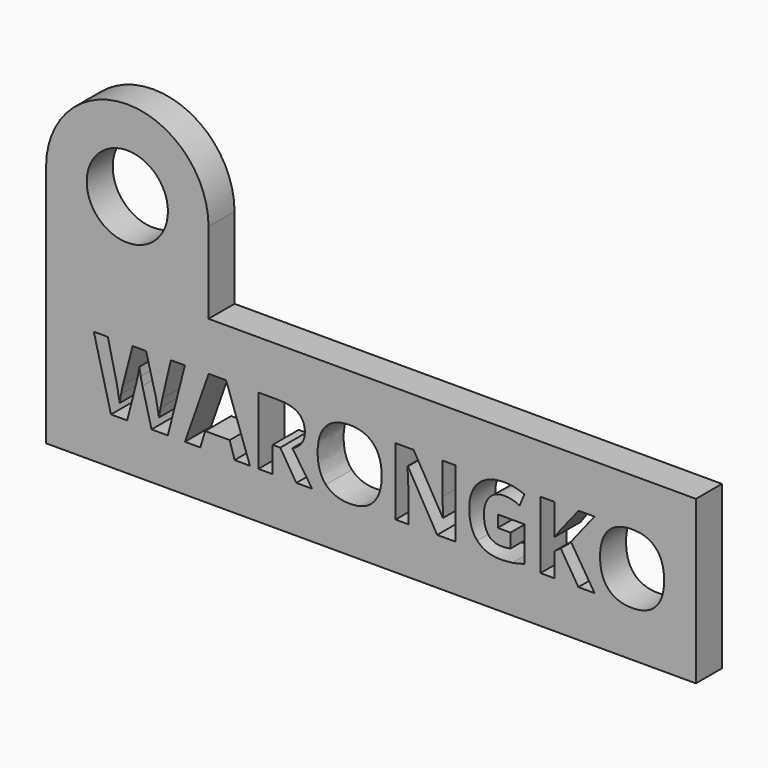
from build123d import *

# Parameters (mm, degrees)
F0_R     = 6.35
F1_DEPTH = 5.08
F2_DEPTH = 25.4


# Not quite as in the source:
# - a feature names something its author has since deleted; it is built from what else it names


with BuildPart() as f1:
    # F0 (on Front) → F1 (new body)
    with BuildSketch(Plane.XZ):
        with BuildLine():
            ThreePointArc((25.4, 38.1), (12.7, 50.8), (0, 38.1))
            ThreePointArc((0, 38.1), (12.7, 25.4), (25.4, 38.1))
        make_face()
        with Locations((12.7, 38.1)):
            Circle(F0_R, mode=Mode.SUBTRACT)
        with BuildLine():
            Line((0, 38.1), (0, 0))
            Line((0, 0), (12.7, 0))
            Line((12.7, 0), (50.8, 0))
            Line((50.8, 0), (101.6, 0))
            Line((101.6, 0), (101.6, 25.4))
            Line((101.6, 25.4), (25.4, 25.4))
            Line((25.4, 25.4), (25.4, 38.1))
            ThreePointArc((25.4, 38.1), (12.7, 25.4), (0, 38.1))
        make_face()
        with BuildLine():
            Line((21.7064113992, 17.7952383145), (19.0291020371, 7.2770728152))
            Line((19.0291020371, 7.2770728152), (16.4899169757, 7.2770728152))
            Line((16.4899169757, 7.2770728152), (15.0649346066, 12.8020448437))
            add(Edge.make_bspline(
                [(15.0649346066, 12.8020448437), (14.9866641696, 13.0967100185), (14.7955922203, 14.0209917975)],
                knots=[0, 0, 0, 1, 1, 1], degree=2))
            add(Edge.make_bspline(
                [(14.7955922203, 14.0209917975), (14.6045202709, 14.9452735764), (14.5768954108, 15.2629594681)],
                knots=[0, 0, 0, 1, 1, 1], degree=2))
            add(Edge.make_bspline(
                [(14.5768954108, 15.2629594681), (14.5331560489, 14.8739093544), (14.360500673, 14.0140855824)],
                knots=[0, 0, 0, 1, 1, 1], degree=2))
            add(Edge.make_bspline(
                [(14.360500673, 14.0140855824), (14.1878452971, 13.1542618105), (14.0934603583, 12.7882324136)],
                knots=[0, 0, 0, 1, 1, 1], degree=2))
            Line((14.0934603583, 12.7882324136), (12.677686276, 7.2770728152))
            Line((12.677686276, 7.2770728152), (10.1454074296, 7.2770728152))
            Line((10.1454074296, 7.2770728152), (7.4611918524, 17.7952383145))
            Line((7.4611918524, 17.7952383145), (9.6550661621, 17.7952383145))
            Line((9.6550661621, 17.7952383145), (11.001778094, 12.0538715482))
            add(Edge.make_bspline(
                [(11.001778094, 12.0538715482), (11.3539950608, 10.4631400183), (11.510535935, 9.2982917489)],
                knots=[0, 0, 0, 1, 1, 1], degree=2))
            add(Edge.make_bspline(
                [(11.510535935, 9.2982917489), (11.5542752969, 9.7080605077), (11.7096651352, 10.5678842797)],
                knots=[0, 0, 0, 1, 1, 1], degree=2))
            add(Edge.make_bspline(
                [(11.7096651352, 10.5678842797), (11.8650549735, 11.4277080516), (12.0008772025, 11.9019348174)],
                knots=[0, 0, 0, 1, 1, 1], degree=2))
            Line((12.0008772025, 11.9019348174), (13.5340569404, 17.7952383145))
            Line((13.5340569404, 17.7952383145), (15.6404525263, 17.7952383145))
            Line((15.6404525263, 17.7952383145), (17.1736322642, 11.9019348174))
            add(Edge.make_bspline(
                [(17.1736322642, 11.9019348174), (17.2749234181, 11.5082805604), (17.425709113, 10.694498222)],
                knots=[0, 0, 0, 1, 1, 1], degree=2))
            add(Edge.make_bspline(
                [(17.425709113, 10.694498222), (17.5764948079, 9.8807158836), (17.654765245, 9.2982917489)],
                knots=[0, 0, 0, 1, 1, 1], degree=2))
            add(Edge.make_bspline(
                [(17.654765245, 9.2982917489), (17.726129467, 9.8599972385), (17.8849724129, 10.6979513295)],
                knots=[0, 0, 0, 1, 1, 1], degree=2))
            add(Edge.make_bspline(
                [(17.8849724129, 10.6979513295), (18.0438153587, 11.5359054205), (18.1727313727, 12.0538715482)],
                knots=[0, 0, 0, 1, 1, 1], degree=2))
            Line((18.1727313727, 12.0538715482), (19.5102350179, 17.7952383145))
            Line((19.5102350179, 17.7952383145), (21.7064113992, 17.7952383145))
        make_face(mode=Mode.SUBTRACT)
        Polygon((31.8723599317, 7.2770728152), (29.4689970993, 7.2770728152), (28.7070113737, 9.7817268014), (24.8717599572, 9.7817268014), (24.1097742317, 7.2770728152), (21.7064113992, 7.2770728152), (25.4196530167, 17.8389776763), (28.1453058841, 17.8389776763), align=None, mode=Mode.SUBTRACT)
        with BuildLine():
            Line((36.6123255178, 11.3126044677), (35.4267586034, 11.3126044677))
            Line((35.4267586034, 11.3126044677), (35.4267586034, 7.2770728152))
            Line((35.4267586034, 7.2770728152), (33.1960511469, 7.2770728152))
            Line((33.1960511469, 7.2770728152), (33.1960511469, 17.7952383145))
            Line((33.1960511469, 17.7952383145), (36.260108551, 17.7952383145))
            add(Edge.make_bspline(
                [(36.260108551, 17.7952383145), (38.4056393554, 17.7952383145), (39.4335143599, 17.0148360154)],
                knots=[0, 0, 0, 1, 1, 1], degree=2))
            add(Edge.make_bspline(
                [(39.4335143599, 17.0148360154), (40.4613893644, 16.2344337164), (40.4613893644, 14.6437021865)],
                knots=[0, 0, 0, 1, 1, 1], degree=2))
            add(Edge.make_bspline(
                [(40.4613893644, 14.6437021865), (40.4613893644, 13.7159673001), (39.9514804876, 12.993116793)],
                knots=[0, 0, 0, 1, 1, 1], degree=2))
            add(Edge.make_bspline(
                [(39.9514804876, 12.993116793), (39.4415716108, 12.2702662859), (38.5046284376, 11.8604975272)],
                knots=[0, 0, 0, 1, 1, 1], degree=2))
            add(Edge.make_bspline(
                [(38.5046284376, 11.8604975272), (40.8803664099, 8.3130050705), (41.5986127736, 7.2770728152)],
                knots=[0, 0, 0, 1, 1, 1], degree=2))
            Line((41.5986127736, 7.2770728152), (39.1238857191, 7.2770728152))
            Line((39.1238857191, 7.2770728152), (36.6123255178, 11.3126044677))
        make_face(mode=Mode.SUBTRACT)
        with BuildLine():
            add(Edge.make_bspline(
                [(51.184439243, 16.5647810023), (52.4689952396, 15.1685745292), (52.4689952396, 12.5511190307)],
                knots=[0, 0, 0, 1, 1, 1], degree=2))
            add(Edge.make_bspline(
                [(52.4689952396, 12.5511190307), (52.4689952396, 9.9382676756), (51.1740799205, 8.5351549875)],
                knots=[0, 0, 0, 1, 1, 1], degree=2))
            add(Edge.make_bspline(
                [(51.1740799205, 8.5351549875), (49.8791646013, 7.1320422994), (47.4619893388, 7.1320422994)],
                knots=[0, 0, 0, 1, 1, 1], degree=2))
            add(Edge.make_bspline(
                [(47.4619893388, 7.1320422994), (45.0448140763, 7.1320422994), (43.7498987572, 8.5351549875)],
                knots=[0, 0, 0, 1, 1, 1], degree=2))
            add(Edge.make_bspline(
                [(43.7498987572, 8.5351549875), (42.454983438, 9.9382676756), (42.454983438, 12.5649314608)],
                knots=[0, 0, 0, 1, 1, 1], degree=2))
            add(Edge.make_bspline(
                [(42.454983438, 12.5649314608), (42.454983438, 15.191595246), (43.7533518647, 16.5762913607)],
                knots=[0, 0, 0, 1, 1, 1], degree=2))
            add(Edge.make_bspline(
                [(43.7533518647, 16.5762913607), (45.0517202914, 17.9609874753), (47.4758017689, 17.9609874753)],
                knots=[0, 0, 0, 1, 1, 1], degree=2))
            add(Edge.make_bspline(
                [(47.4758017689, 17.9609874753), (49.8998832464, 17.9609874753), (51.184439243, 16.5647810023)],
                knots=[0, 0, 0, 1, 1, 1], degree=2))
        make_face(mode=Mode.SUBTRACT)
        with BuildLine():
            Line((63.9793536324, 17.7952383145), (63.9793536324, 7.2770728152))
            Line((63.9793536324, 7.2770728152), (61.1455033961, 7.2770728152))
            Line((61.1455033961, 7.2770728152), (56.5689848991, 15.2330325362))
            Line((56.5689848991, 15.2330325362), (56.5045268921, 15.2330325362))
            add(Edge.make_bspline(
                [(56.5045268921, 15.2330325362), (56.6426511928, 13.1266369504), (56.6426511928, 12.2265269241)],
                knots=[0, 0, 0, 1, 1, 1], degree=2))
            Line((56.6426511928, 12.2265269241), (56.6426511928, 7.2770728152))
            Line((56.6426511928, 7.2770728152), (54.6490571192, 7.2770728152))
            Line((54.6490571192, 7.2770728152), (54.6490571192, 17.7952383145))
            Line((54.6490571192, 17.7952383145), (57.4621887104, 17.7952383145))
            Line((57.4621887104, 17.7952383145), (62.0294989206, 9.9175490305))
            Line((62.0294989206, 9.9175490305), (62.0801444976, 9.9175490305))
            add(Edge.make_bspline(
                [(62.0801444976, 9.9175490305), (61.9719471287, 11.9686948961), (61.9719471287, 12.8158572738)],
                knots=[0, 0, 0, 1, 1, 1], degree=2))
            Line((61.9719471287, 12.8158572738), (61.9719471287, 17.7952383145))
            Line((61.9719471287, 17.7952383145), (63.9793536324, 17.7952383145))
        make_face(mode=Mode.SUBTRACT)
        with BuildLine():
            Line((70.6185283533, 11.3264168977), (70.6185283533, 13.1841887423))
            Line((70.6185283533, 13.1841887423), (74.7921843065, 13.1841887423))
            Line((74.7921843065, 13.1841887423), (74.7921843065, 7.7305809359))
            add(Edge.make_bspline(
                [(74.7921843065, 7.7305809359), (73.7769706963, 7.3990826141), (72.8814648133, 7.2655624568)],
                knots=[0, 0, 0, 1, 1, 1], degree=2))
            add(Edge.make_bspline(
                [(72.8814648133, 7.2655624568), (71.9859589304, 7.1320422994), (71.0513178289, 7.1320422994)],
                knots=[0, 0, 0, 1, 1, 1], degree=2))
            add(Edge.make_bspline(
                [(71.0513178289, 7.1320422994), (68.6709757132, 7.1320422994), (67.4151956126, 8.53170188)],
                knots=[0, 0, 0, 1, 1, 1], degree=2))
            add(Edge.make_bspline(
                [(67.4151956126, 8.53170188), (66.159415512, 9.9313614605), (66.159415512, 12.5511190307)],
                knots=[0, 0, 0, 1, 1, 1], degree=2))
            add(Edge.make_bspline(
                [(66.159415512, 12.5511190307), (66.159415512, 15.0972103072), (67.6166268845, 16.5210416404)],
                knots=[0, 0, 0, 1, 1, 1], degree=2))
            add(Edge.make_bspline(
                [(67.6166268845, 16.5210416404), (69.073838257, 17.9448729736), (71.6544606086, 17.9448729736)],
                knots=[0, 0, 0, 1, 1, 1], degree=2))
            add(Edge.make_bspline(
                [(71.6544606086, 17.9448729736), (73.2751190703, 17.9448729736), (74.7783718764, 17.2979908319)],
                knots=[0, 0, 0, 1, 1, 1], degree=2))
            Line((74.7783718764, 17.2979908319), (74.0371047959, 15.513885281))
            add(Edge.make_bspline(
                [(74.0371047959, 15.513885281), (72.8860689567, 16.0894032007), (71.6406481786, 16.0894032007)],
                knots=[0, 0, 0, 1, 1, 1], degree=2))
            add(Edge.make_bspline(
                [(71.6406481786, 16.0894032007), (70.1949471644, 16.0894032007), (69.32476407, 15.1179289523)],
                knots=[0, 0, 0, 1, 1, 1], degree=2))
            add(Edge.make_bspline(
                [(69.32476407, 15.1179289523), (68.4545809755, 14.146454704), (68.4545809755, 12.5073796688)],
                knots=[0, 0, 0, 1, 1, 1], degree=2))
            add(Edge.make_bspline(
                [(68.4545809755, 12.5073796688), (68.4545809755, 10.79463834), (69.1555618016, 9.892226242)],
                knots=[0, 0, 0, 1, 1, 1], degree=2))
            add(Edge.make_bspline(
                [(69.1555618016, 9.892226242), (69.8565426277, 8.989814144), (71.1940462729, 8.989814144)],
                knots=[0, 0, 0, 1, 1, 1], degree=2))
            add(Edge.make_bspline(
                [(71.1940462729, 8.989814144), (71.8938760632, 8.989814144), (72.6121224269, 9.1325425881)],
                knots=[0, 0, 0, 1, 1, 1], degree=2))
            Line((72.6121224269, 9.1325425881), (72.6121224269, 11.3264168977))
            Line((72.6121224269, 11.3264168977), (70.6185283533, 11.3264168977))
        make_face(mode=Mode.SUBTRACT)
        Polygon((82.057522524, 13.1404493804), (85.7546496397, 7.2770728152), (83.2223707933, 7.2770728152), (80.4667909941, 11.7085607964), (79.5252436776, 11.0317517229), (79.5252436776, 7.2770728152), (77.2945362211, 7.2770728152), (77.2945362211, 17.7952383145), (79.5252436776, 17.7952383145), (79.5252436776, 12.9816064346), (80.4023329871, 14.2201209977), (83.2522977251, 17.7952383145), (85.7270247796, 17.7952383145), align=None, mode=Mode.SUBTRACT)
        with BuildLine():
            add(Edge.make_bspline(
                [(95.3404761092, 16.5647810023), (96.6250321058, 15.1685745292), (96.6250321058, 12.5511190307)],
                knots=[0, 0, 0, 1, 1, 1], degree=2))
            add(Edge.make_bspline(
                [(96.6250321058, 12.5511190307), (96.6250321058, 9.9382676756), (95.3301167866, 8.5351549875)],
                knots=[0, 0, 0, 1, 1, 1], degree=2))
            add(Edge.make_bspline(
                [(95.3301167866, 8.5351549875), (94.0352014675, 7.1320422994), (91.618026205, 7.1320422994)],
                knots=[0, 0, 0, 1, 1, 1], degree=2))
            add(Edge.make_bspline(
                [(91.618026205, 7.1320422994), (89.2008509425, 7.1320422994), (87.9059356233, 8.5351549875)],
                knots=[0, 0, 0, 1, 1, 1], degree=2))
            add(Edge.make_bspline(
                [(87.9059356233, 8.5351549875), (86.6110203041, 9.9382676756), (86.6110203041, 12.5649314608)],
                knots=[0, 0, 0, 1, 1, 1], degree=2))
            add(Edge.make_bspline(
                [(86.6110203041, 12.5649314608), (86.6110203041, 15.191595246), (87.9093887308, 16.5762913607)],
                knots=[0, 0, 0, 1, 1, 1], degree=2))
            add(Edge.make_bspline(
                [(87.9093887308, 16.5762913607), (89.2077571575, 17.9609874753), (91.6318386351, 17.9609874753)],
                knots=[0, 0, 0, 1, 1, 1], degree=2))
            add(Edge.make_bspline(
                [(91.6318386351, 17.9609874753), (94.0559201126, 17.9609874753), (95.3404761092, 16.5647810023)],
                knots=[0, 0, 0, 1, 1, 1], degree=2))
        make_face(mode=Mode.SUBTRACT)
    extrude(amount=F1_DEPTH)

    # F0 (on Front) → F2 (cut)
    with BuildSketch(Plane.XZ):
        with BuildLine():
            Line((0, 38.1), (0, 0))
            Line((0, 0), (12.7, 0))
            Line((12.7, 0), (50.8, 0))
            Line((50.8, 0), (101.6, 0))
            Line((101.6, 0), (101.6, 25.4))
            Line((101.6, 25.4), (25.4, 25.4))
            Line((25.4, 25.4), (25.4, 38.1))
            ThreePointArc((25.4, 38.1), (12.7, 25.4), (0, 38.1))
        make_face()
        with BuildLine():
            Line((21.7064113992, 17.7952383145), (19.0291020371, 7.2770728152))
            Line((19.0291020371, 7.2770728152), (16.4899169757, 7.2770728152))
            Line((16.4899169757, 7.2770728152), (15.0649346066, 12.8020448437))
            add(Edge.make_bspline(
                [(15.0649346066, 12.8020448437), (14.9866641696, 13.0967100185), (14.7955922203, 14.0209917975)],
                knots=[0, 0, 0, 1, 1, 1], degree=2))
            add(Edge.make_bspline(
                [(14.7955922203, 14.0209917975), (14.6045202709, 14.9452735764), (14.5768954108, 15.2629594681)],
                knots=[0, 0, 0, 1, 1, 1], degree=2))
            add(Edge.make_bspline(
                [(14.5768954108, 15.2629594681), (14.5331560489, 14.8739093544), (14.360500673, 14.0140855824)],
                knots=[0, 0, 0, 1, 1, 1], degree=2))
            add(Edge.make_bspline(
                [(14.360500673, 14.0140855824), (14.1878452971, 13.1542618105), (14.0934603583, 12.7882324136)],
                knots=[0, 0, 0, 1, 1, 1], degree=2))
            Line((14.0934603583, 12.7882324136), (12.677686276, 7.2770728152))
            Line((12.677686276, 7.2770728152), (10.1454074296, 7.2770728152))
            Line((10.1454074296, 7.2770728152), (7.4611918524, 17.7952383145))
            Line((7.4611918524, 17.7952383145), (9.6550661621, 17.7952383145))
            Line((9.6550661621, 17.7952383145), (11.001778094, 12.0538715482))
            add(Edge.make_bspline(
                [(11.001778094, 12.0538715482), (11.3539950608, 10.4631400183), (11.510535935, 9.2982917489)],
                knots=[0, 0, 0, 1, 1, 1], degree=2))
            add(Edge.make_bspline(
                [(11.510535935, 9.2982917489), (11.5542752969, 9.7080605077), (11.7096651352, 10.5678842797)],
                knots=[0, 0, 0, 1, 1, 1], degree=2))
            add(Edge.make_bspline(
                [(11.7096651352, 10.5678842797), (11.8650549735, 11.4277080516), (12.0008772025, 11.9019348174)],
                knots=[0, 0, 0, 1, 1, 1], degree=2))
            Line((12.0008772025, 11.9019348174), (13.5340569404, 17.7952383145))
            Line((13.5340569404, 17.7952383145), (15.6404525263, 17.7952383145))
            Line((15.6404525263, 17.7952383145), (17.1736322642, 11.9019348174))
            add(Edge.make_bspline(
                [(17.1736322642, 11.9019348174), (17.2749234181, 11.5082805604), (17.425709113, 10.694498222)],
                knots=[0, 0, 0, 1, 1, 1], degree=2))
            add(Edge.make_bspline(
                [(17.425709113, 10.694498222), (17.5764948079, 9.8807158836), (17.654765245, 9.2982917489)],
                knots=[0, 0, 0, 1, 1, 1], degree=2))
            add(Edge.make_bspline(
                [(17.654765245, 9.2982917489), (17.726129467, 9.8599972385), (17.8849724129, 10.6979513295)],
                knots=[0, 0, 0, 1, 1, 1], degree=2))
            add(Edge.make_bspline(
                [(17.8849724129, 10.6979513295), (18.0438153587, 11.5359054205), (18.1727313727, 12.0538715482)],
                knots=[0, 0, 0, 1, 1, 1], degree=2))
            Line((18.1727313727, 12.0538715482), (19.5102350179, 17.7952383145))
            Line((19.5102350179, 17.7952383145), (21.7064113992, 17.7952383145))
        make_face(mode=Mode.SUBTRACT)
        Polygon((31.8723599317, 7.2770728152), (29.4689970993, 7.2770728152), (28.7070113737, 9.7817268014), (24.8717599572, 9.7817268014), (24.1097742317, 7.2770728152), (21.7064113992, 7.2770728152), (25.4196530167, 17.8389776763), (28.1453058841, 17.8389776763), align=None, mode=Mode.SUBTRACT)
        with BuildLine():
            Line((36.6123255178, 11.3126044677), (35.4267586034, 11.3126044677))
            Line((35.4267586034, 11.3126044677), (35.4267586034, 7.2770728152))
            Line((35.4267586034, 7.2770728152), (33.1960511469, 7.2770728152))
            Line((33.1960511469, 7.2770728152), (33.1960511469, 17.7952383145))
            Line((33.1960511469, 17.7952383145), (36.260108551, 17.7952383145))
            add(Edge.make_bspline(
                [(36.260108551, 17.7952383145), (38.4056393554, 17.7952383145), (39.4335143599, 17.0148360154)],
                knots=[0, 0, 0, 1, 1, 1], degree=2))
            add(Edge.make_bspline(
                [(39.4335143599, 17.0148360154), (40.4613893644, 16.2344337164), (40.4613893644, 14.6437021865)],
                knots=[0, 0, 0, 1, 1, 1], degree=2))
            add(Edge.make_bspline(
                [(40.4613893644, 14.6437021865), (40.4613893644, 13.7159673001), (39.9514804876, 12.993116793)],
                knots=[0, 0, 0, 1, 1, 1], degree=2))
            add(Edge.make_bspline(
                [(39.9514804876, 12.993116793), (39.4415716108, 12.2702662859), (38.5046284376, 11.8604975272)],
                knots=[0, 0, 0, 1, 1, 1], degree=2))
            add(Edge.make_bspline(
                [(38.5046284376, 11.8604975272), (40.8803664099, 8.3130050705), (41.5986127736, 7.2770728152)],
                knots=[0, 0, 0, 1, 1, 1], degree=2))
            Line((41.5986127736, 7.2770728152), (39.1238857191, 7.2770728152))
            Line((39.1238857191, 7.2770728152), (36.6123255178, 11.3126044677))
        make_face(mode=Mode.SUBTRACT)
        with BuildLine():
            add(Edge.make_bspline(
                [(51.184439243, 16.5647810023), (52.4689952396, 15.1685745292), (52.4689952396, 12.5511190307)],
                knots=[0, 0, 0, 1, 1, 1], degree=2))
            add(Edge.make_bspline(
                [(52.4689952396, 12.5511190307), (52.4689952396, 9.9382676756), (51.1740799205, 8.5351549875)],
                knots=[0, 0, 0, 1, 1, 1], degree=2))
            add(Edge.make_bspline(
                [(51.1740799205, 8.5351549875), (49.8791646013, 7.1320422994), (47.4619893388, 7.1320422994)],
                knots=[0, 0, 0, 1, 1, 1], degree=2))
            add(Edge.make_bspline(
                [(47.4619893388, 7.1320422994), (45.0448140763, 7.1320422994), (43.7498987572, 8.5351549875)],
                knots=[0, 0, 0, 1, 1, 1], degree=2))
            add(Edge.make_bspline(
                [(43.7498987572, 8.5351549875), (42.454983438, 9.9382676756), (42.454983438, 12.5649314608)],
                knots=[0, 0, 0, 1, 1, 1], degree=2))
            add(Edge.make_bspline(
                [(42.454983438, 12.5649314608), (42.454983438, 15.191595246), (43.7533518647, 16.5762913607)],
                knots=[0, 0, 0, 1, 1, 1], degree=2))
            add(Edge.make_bspline(
                [(43.7533518647, 16.5762913607), (45.0517202914, 17.9609874753), (47.4758017689, 17.9609874753)],
                knots=[0, 0, 0, 1, 1, 1], degree=2))
            add(Edge.make_bspline(
                [(47.4758017689, 17.9609874753), (49.8998832464, 17.9609874753), (51.184439243, 16.5647810023)],
                knots=[0, 0, 0, 1, 1, 1], degree=2))
        make_face(mode=Mode.SUBTRACT)
        with BuildLine():
            Line((63.9793536324, 17.7952383145), (63.9793536324, 7.2770728152))
            Line((63.9793536324, 7.2770728152), (61.1455033961, 7.2770728152))
            Line((61.1455033961, 7.2770728152), (56.5689848991, 15.2330325362))
            Line((56.5689848991, 15.2330325362), (56.5045268921, 15.2330325362))
            add(Edge.make_bspline(
                [(56.5045268921, 15.2330325362), (56.6426511928, 13.1266369504), (56.6426511928, 12.2265269241)],
                knots=[0, 0, 0, 1, 1, 1], degree=2))
            Line((56.6426511928, 12.2265269241), (56.6426511928, 7.2770728152))
            Line((56.6426511928, 7.2770728152), (54.6490571192, 7.2770728152))
            Line((54.6490571192, 7.2770728152), (54.6490571192, 17.7952383145))
            Line((54.6490571192, 17.7952383145), (57.4621887104, 17.7952383145))
            Line((57.4621887104, 17.7952383145), (62.0294989206, 9.9175490305))
            Line((62.0294989206, 9.9175490305), (62.0801444976, 9.9175490305))
            add(Edge.make_bspline(
                [(62.0801444976, 9.9175490305), (61.9719471287, 11.9686948961), (61.9719471287, 12.8158572738)],
                knots=[0, 0, 0, 1, 1, 1], degree=2))
            Line((61.9719471287, 12.8158572738), (61.9719471287, 17.7952383145))
            Line((61.9719471287, 17.7952383145), (63.9793536324, 17.7952383145))
        make_face(mode=Mode.SUBTRACT)
        with BuildLine():
            Line((70.6185283533, 11.3264168977), (70.6185283533, 13.1841887423))
            Line((70.6185283533, 13.1841887423), (74.7921843065, 13.1841887423))
            Line((74.7921843065, 13.1841887423), (74.7921843065, 7.7305809359))
            add(Edge.make_bspline(
                [(74.7921843065, 7.7305809359), (73.7769706963, 7.3990826141), (72.8814648133, 7.2655624568)],
                knots=[0, 0, 0, 1, 1, 1], degree=2))
            add(Edge.make_bspline(
                [(72.8814648133, 7.2655624568), (71.9859589304, 7.1320422994), (71.0513178289, 7.1320422994)],
                knots=[0, 0, 0, 1, 1, 1], degree=2))
            add(Edge.make_bspline(
                [(71.0513178289, 7.1320422994), (68.6709757132, 7.1320422994), (67.4151956126, 8.53170188)],
                knots=[0, 0, 0, 1, 1, 1], degree=2))
            add(Edge.make_bspline(
                [(67.4151956126, 8.53170188), (66.159415512, 9.9313614605), (66.159415512, 12.5511190307)],
                knots=[0, 0, 0, 1, 1, 1], degree=2))
            add(Edge.make_bspline(
                [(66.159415512, 12.5511190307), (66.159415512, 15.0972103072), (67.6166268845, 16.5210416404)],
                knots=[0, 0, 0, 1, 1, 1], degree=2))
            add(Edge.make_bspline(
                [(67.6166268845, 16.5210416404), (69.073838257, 17.9448729736), (71.6544606086, 17.9448729736)],
                knots=[0, 0, 0, 1, 1, 1], degree=2))
            add(Edge.make_bspline(
                [(71.6544606086, 17.9448729736), (73.2751190703, 17.9448729736), (74.7783718764, 17.2979908319)],
                knots=[0, 0, 0, 1, 1, 1], degree=2))
            Line((74.7783718764, 17.2979908319), (74.0371047959, 15.513885281))
            add(Edge.make_bspline(
                [(74.0371047959, 15.513885281), (72.8860689567, 16.0894032007), (71.6406481786, 16.0894032007)],
                knots=[0, 0, 0, 1, 1, 1], degree=2))
            add(Edge.make_bspline(
                [(71.6406481786, 16.0894032007), (70.1949471644, 16.0894032007), (69.32476407, 15.1179289523)],
                knots=[0, 0, 0, 1, 1, 1], degree=2))
            add(Edge.make_bspline(
                [(69.32476407, 15.1179289523), (68.4545809755, 14.146454704), (68.4545809755, 12.5073796688)],
                knots=[0, 0, 0, 1, 1, 1], degree=2))
            add(Edge.make_bspline(
                [(68.4545809755, 12.5073796688), (68.4545809755, 10.79463834), (69.1555618016, 9.892226242)],
                knots=[0, 0, 0, 1, 1, 1], degree=2))
            add(Edge.make_bspline(
                [(69.1555618016, 9.892226242), (69.8565426277, 8.989814144), (71.1940462729, 8.989814144)],
                knots=[0, 0, 0, 1, 1, 1], degree=2))
            add(Edge.make_bspline(
                [(71.1940462729, 8.989814144), (71.8938760632, 8.989814144), (72.6121224269, 9.1325425881)],
                knots=[0, 0, 0, 1, 1, 1], degree=2))
            Line((72.6121224269, 9.1325425881), (72.6121224269, 11.3264168977))
            Line((72.6121224269, 11.3264168977), (70.6185283533, 11.3264168977))
        make_face(mode=Mode.SUBTRACT)
        Polygon((82.057522524, 13.1404493804), (85.7546496397, 7.2770728152), (83.2223707933, 7.2770728152), (80.4667909941, 11.7085607964), (79.5252436776, 11.0317517229), (79.5252436776, 7.2770728152), (77.2945362211, 7.2770728152), (77.2945362211, 17.7952383145), (79.5252436776, 17.7952383145), (79.5252436776, 12.9816064346), (80.4023329871, 14.2201209977), (83.2522977251, 17.7952383145), (85.7270247796, 17.7952383145), align=None, mode=Mode.SUBTRACT)
        with BuildLine():
            add(Edge.make_bspline(
                [(95.3404761092, 16.5647810023), (96.6250321058, 15.1685745292), (96.6250321058, 12.5511190307)],
                knots=[0, 0, 0, 1, 1, 1], degree=2))
            add(Edge.make_bspline(
                [(96.6250321058, 12.5511190307), (96.6250321058, 9.9382676756), (95.3301167866, 8.5351549875)],
                knots=[0, 0, 0, 1, 1, 1], degree=2))
            add(Edge.make_bspline(
                [(95.3301167866, 8.5351549875), (94.0352014675, 7.1320422994), (91.618026205, 7.1320422994)],
                knots=[0, 0, 0, 1, 1, 1], degree=2))
            add(Edge.make_bspline(
                [(91.618026205, 7.1320422994), (89.2008509425, 7.1320422994), (87.9059356233, 8.5351549875)],
                knots=[0, 0, 0, 1, 1, 1], degree=2))
            add(Edge.make_bspline(
                [(87.9059356233, 8.5351549875), (86.6110203041, 9.9382676756), (86.6110203041, 12.5649314608)],
                knots=[0, 0, 0, 1, 1, 1], degree=2))
            add(Edge.make_bspline(
                [(86.6110203041, 12.5649314608), (86.6110203041, 15.191595246), (87.9093887308, 16.5762913607)],
                knots=[0, 0, 0, 1, 1, 1], degree=2))
            add(Edge.make_bspline(
                [(87.9093887308, 16.5762913607), (89.2077571575, 17.9609874753), (91.6318386351, 17.9609874753)],
                knots=[0, 0, 0, 1, 1, 1], degree=2))
            add(Edge.make_bspline(
                [(91.6318386351, 17.9609874753), (94.0559201126, 17.9609874753), (95.3404761092, 16.5647810023)],
                knots=[0, 0, 0, 1, 1, 1], degree=2))
        make_face(mode=Mode.SUBTRACT)
        with BuildLine():
            ThreePointArc((25.4, 38.1), (12.7, 50.8), (0, 38.1))
            ThreePointArc((0, 38.1), (12.7, 25.4), (25.4, 38.1))
        make_face()
        with Locations((12.7, 38.1)):
            Circle(F0_R, mode=Mode.SUBTRACT)
    extrude(amount=-F2_DEPTH, mode=Mode.SUBTRACT)


solid = f1.part
